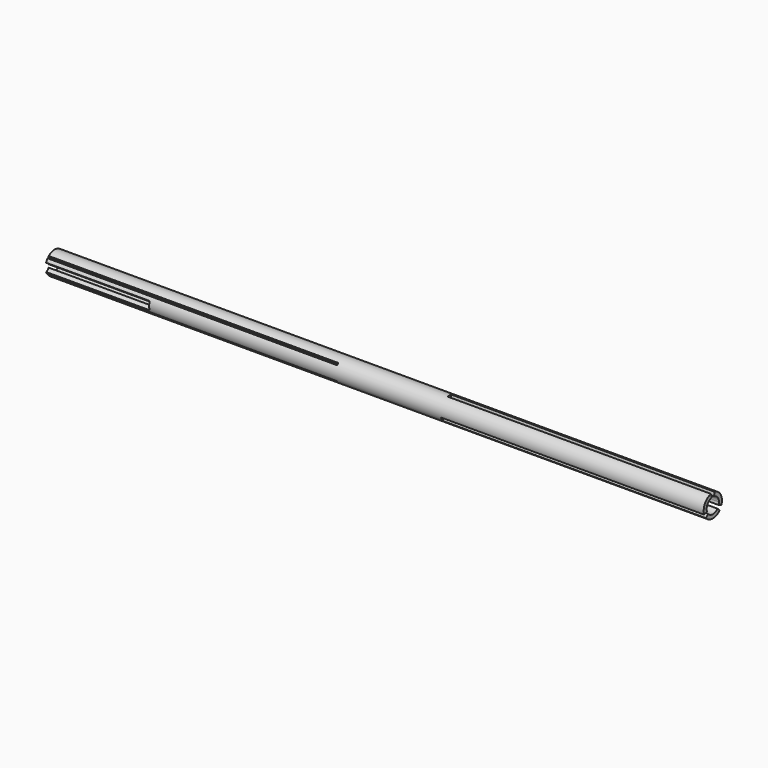
from build123d import *

# Parameters (mm, degrees)
F0_R     = 11
F1_DEPTH = 635
F3_DEPTH = 254
F4_R     = 7.4
F5_DEPTH = 380
F7_DEPTH = 279.4
F8_DEPTH = 100


with BuildPart() as f1:
    # F0 (on Right) → F1 (new body)
    with BuildSketch(Plane.YZ):
        Circle(F0_R)
    extrude(amount=F1_DEPTH)

    # F2 (on face) → F3 (cut)
    with BuildSketch(Plane.YZ.offset(635)):
        with BuildLine():
            ThreePointArc((0, 7.39), (0.724346667, 7.3544151301), (1.4417174797, 7.2480032222))
            Line((1.4417174797, 7.2480032222), (2.1459935422, 10.7886380844))
            ThreePointArc((2.1459935422, 10.7886380844), (0, 11), (-2.1459935422, 10.7886380844))
            Line((-2.1459935422, 10.7886380844), (-1.4417174797, 7.2480032222))
            ThreePointArc((-1.4417174797, 7.2480032222), (-0.724346667, 7.3544151301), (0, 7.39))
        make_face()
        with BuildLine():
            Line((-6.997813657, -2.3754376486), (0, 0))
            Line((0, 0), (-1.4417174797, 7.2480032222))
            ThreePointArc((-1.4417174797, 7.2480032222), (-6.399927734, 3.695), (-6.997813657, -2.3754376486))
        make_face()
        with BuildLine():
            Line((-5.5560961773, -4.8725655736), (0, 0))
            Line((0, 0), (-6.997813657, -2.3754376486))
            ThreePointArc((-6.997813657, -2.3754376486), (-6.399927734, -3.695), (-5.5560961773, -4.8725655736))
        make_face()
        with BuildLine():
            Line((5.5560961773, -4.8725655736), (0, 0))
            Line((0, 0), (-5.5560961773, -4.8725655736))
            ThreePointArc((-5.5560961773, -4.8725655736), (0, -7.39), (5.5560961773, -4.8725655736))
        make_face()
        with BuildLine():
            ThreePointArc((5.5560961773, -4.8725655736), (6.399927734, -3.695), (6.997813657, -2.3754376486))
            Line((6.997813657, -2.3754376486), (0, 0))
            Line((0, 0), (5.5560961773, -4.8725655736))
        make_face()
        with BuildLine():
            ThreePointArc((6.997813657, -2.3754376486), (7.2912942241, -1.2037975484), (7.39, 0))
            ThreePointArc((7.39, 0), (5.7125472504, 4.68816637), (1.4417174797, 7.2480032222))
            Line((1.4417174797, 7.2480032222), (0, 0))
            Line((0, 0), (6.997813657, -2.3754376486))
        make_face()
        with BuildLine():
            Line((0, 0), (1.4417174797, 7.2480032222))
            ThreePointArc((1.4417174797, 7.2480032222), (0.724346667, 7.3544151301), (0, 7.39))
            Line((0, 7.39), (0, 0))
        make_face()
        with BuildLine():
            Line((0, 0), (0, 7.39))
            ThreePointArc((0, 7.39), (-0.724346667, 7.3544151301), (-1.4417174797, 7.2480032222))
            Line((-1.4417174797, 7.2480032222), (0, 0))
        make_face()
        with BuildLine():
            ThreePointArc((-5.5560961773, -4.8725655736), (-6.399927734, -3.695), (-6.997813657, -2.3754376486))
            Line((-6.997813657, -2.3754376486), (-10.4162314244, -3.5358341183))
            ThreePointArc((-10.4162314244, -3.5358341183), (-9.5262794416, -5.5), (-8.2702378823, -7.2528039661))
            Line((-8.2702378823, -7.2528039661), (-5.5560961773, -4.8725655736))
        make_face()
        with BuildLine():
            Line((10.4162314244, -3.5358341183), (6.997813657, -2.3754376486))
            ThreePointArc((6.997813657, -2.3754376486), (6.399927734, -3.695), (5.5560961773, -4.8725655736))
            Line((5.5560961773, -4.8725655736), (8.2702378823, -7.2528039661))
            ThreePointArc((8.2702378823, -7.2528039661), (9.5262794416, -5.5), (10.4162314244, -3.5358341183))
        make_face()
    extrude(amount=-F3_DEPTH, mode=Mode.SUBTRACT)

    # F4 (on face) → F5 (cut)
    with BuildSketch(Plane(origin=(0, 0, 0), x_dir=(0, -1, 0), z_dir=(-1, 0, 0))):
        Circle(F4_R)
    extrude(amount=-F5_DEPTH, mode=Mode.SUBTRACT)

    # F6 (on face) → F7 (cut)
    with BuildSketch(Plane(origin=(0, 0, 0), x_dir=(0, -1, 0), z_dir=(-1, 0, 0))):
        with BuildLine():
            Line((7.1172844619, 8.3871486149), (7.1172844619, 6.972222589))
            Line((7.1172844619, 6.972222589), (8.5081203665, 6.972222589))
            ThreePointArc((8.5081203665, 6.972222589), (7.8446684396, 7.7111073831), (7.1172844619, 8.3871486149))
        make_face()
        with BuildLine():
            ThreePointArc((-9.0388867634, -6.2688536495), (-8.2077799909, -7.3234109281), (-7.2543820773, -8.2688536495))
            Line((-7.2543820773, -8.2688536495), (-7.2051168904, -8.2688536495))
            Line((-7.2051168904, -8.2688536495), (-7.2051168904, -6.2688536495))
            Line((-7.2051168904, -6.2688536495), (-9.0388867634, -6.2688536495))
        make_face()
        with BuildLine():
            ThreePointArc((7.2543820773, -8.2688536495), (8.2077799909, -7.3234109281), (9.0388867634, -6.2688536495))
            Line((9.0388867634, -6.2688536495), (7.1172844619, -6.2688536495))
            Line((7.1172844619, -6.2688536495), (7.1172844619, -8.2688536495))
            Line((7.1172844619, -8.2688536495), (7.2543820773, -8.2688536495))
        make_face()
        with BuildLine():
            Line((-7.2051168904, 6.972222589), (-7.2051168904, 8.3118163235))
            ThreePointArc((-7.2051168904, 8.3118163235), (-7.8851178885, 7.6697402749), (-8.5081203665, 6.972222589))
            Line((-8.5081203665, 6.972222589), (-7.2051168904, 6.972222589))
        make_face()
    extrude(amount=-F7_DEPTH, mode=Mode.SUBTRACT)

    # F6 (on face) → F8 (cut)
    with BuildSketch(Plane(origin=(0, 0, 0), x_dir=(0, -1, 0), z_dir=(-1, 0, 0))):
        with BuildLine():
            ThreePointArc((11, 0), (10.8166538264, 2), (10.2727272727, 3.9333286641))
            ThreePointArc((10.2727272727, 3.9333286641), (8.4387429279, 3.0724521494), (7.2618181818, 1.4233751066))
            ThreePointArc((7.2618181818, 1.4233751066), (7.3653735325, 0.7150333749), (7.4, 0))
            ThreePointArc((7.4, 0), (7.3653735325, -0.7150333749), (7.2618181818, -1.4233751066))
            ThreePointArc((7.2618181818, -1.4233751066), (8.4387429279, -3.0724521494), (10.2727272727, -3.9333286641))
            ThreePointArc((10.2727272727, -3.9333286641), (10.8166538264, -2), (11, 0))
        make_face()
        with BuildLine():
            ThreePointArc((-7.2618181818, -1.4233751066), (-7.4, 0), (-7.2618181818, 1.4233751066))
            ThreePointArc((-7.2618181818, 1.4233751066), (-8.4387429279, 3.0724521494), (-10.2727272727, 3.9333286641))
            ThreePointArc((-10.2727272727, 3.9333286641), (-11, 0), (-10.2727272727, -3.9333286641))
            ThreePointArc((-10.2727272727, -3.9333286641), (-8.4387429279, -3.0724521494), (-7.2618181818, -1.4233751066))
        make_face()
    extrude(amount=-F8_DEPTH, mode=Mode.SUBTRACT)


solid = f1.part
